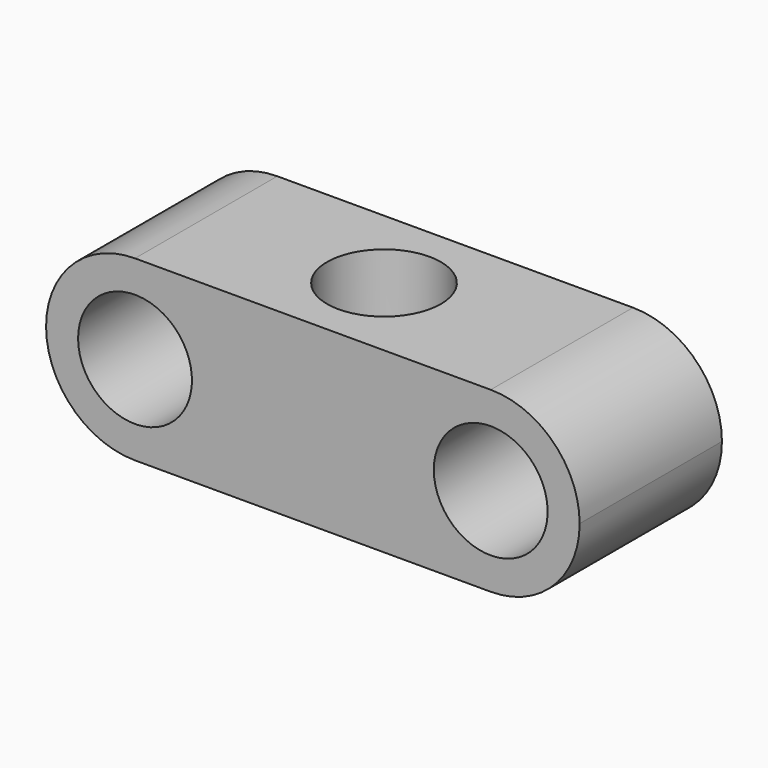
from build123d import *

# Parameters (mm, degrees)
F0_W     = 23.8125
F0_H     = 7.9375
F0_R     = 2.54
F1_DEPTH = 7.9375
F3_DEPTH = 7.9375
F4_R     = 3.96874


# Not quite as in the source:
# - a fillet or chamfer is up to 0.001 mm smaller than in the source, because OpenCascade refuses the exact size


with BuildPart() as f1:
    # F0 (on Top) → F1 (new body)
    with BuildSketch(Plane.XY):
        Rectangle(F0_W, F0_H)
        Circle(F0_R, mode=Mode.SUBTRACT)
    extrude(amount=F1_DEPTH)

    # F2 (on face) → F3 (cut, through all)
    with BuildSketch(Plane.XZ.offset(3.96875)):
        with BuildLine():
            ThreePointArc((-5.3975, 3.96875), (-7.9375, 6.50875), (-10.4775, 3.96875))
            Line((-10.4775, 3.96875), (-7.9375, 3.96875))
            Line((-7.9375, 3.96875), (-5.3975, 3.96875))
        make_face()
        with BuildLine():
            ThreePointArc((10.4775, 3.96875), (7.9375, 6.50875), (5.3975, 3.96875))
            Line((5.3975, 3.96875), (7.9375, 3.96875))
            Line((7.9375, 3.96875), (10.4775, 3.96875))
        make_face()
        with BuildLine():
            Line((7.9375, 3.96875), (5.3975, 3.96875))
            ThreePointArc((5.3975, 3.96875), (7.9375, 1.42875), (10.4775, 3.96875))
            Line((10.4775, 3.96875), (7.9375, 3.96875))
        make_face()
        with BuildLine():
            Line((-7.9375, 3.96875), (-10.4775, 3.96875))
            ThreePointArc((-10.4775, 3.96875), (-7.9375, 1.42875), (-5.3975, 3.96875))
            Line((-5.3975, 3.96875), (-7.9375, 3.96875))
        make_face()
    extrude(amount=-F3_DEPTH, mode=Mode.SUBTRACT)

    # F4 (radius 3.96875 in the source; OpenCascade refuses exactly that, so slightly less here)
    f4_edges = [f1.edges().sort_by_distance(p)[0] for p in [
        (11.90625, 0, 7.9375),
        (11.90625, 0, 0),
        (-11.90625, 0, 7.9375),
        (-11.90625, 0, 0),
    ]]
    fillet(f4_edges, radius=F4_R)


solid = f1.part
